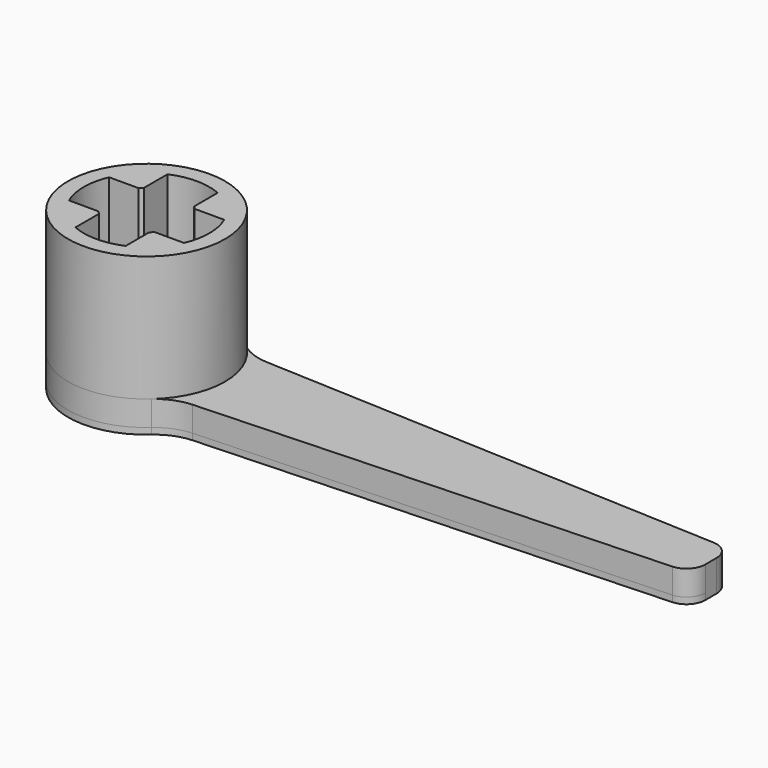
from build123d import *

# Parameters (mm, degrees)
F0_R     = 12.5
F1_DEPTH = 20
F3_DEPTH = 5
F4_DEPTH = 4
F5_R     = 8
F6_R     = 3


with BuildPart() as f1:
    # F0 (on Top) → F1 (new body)
    with BuildSketch(Plane.XY):
        Circle(F0_R)
        with BuildLine():
            ThreePointArc((-9.1651513899, -4), (-10, 0), (-9.1651513899, 4))
            Line((-9.1651513899, 4), (-4.472135955, 4))
            ThreePointArc((-4.472135955, 4), (-4.2426406871, 4.2426406871), (-4, 4.472135955))
            Line((-4, 4.472135955), (-4, 9.1651513899))
            ThreePointArc((-4, 9.1651513899), (0, 10), (4, 9.1651513899))
            Line((4, 9.1651513899), (4, 4.472135955))
            ThreePointArc((4, 4.472135955), (4.2426406871, 4.2426406871), (4.472135955, 4))
            Line((4.472135955, 4), (9.1651513899, 4))
            ThreePointArc((9.1651513899, 4), (10, 0), (9.1651513899, -4))
            Line((9.1651513899, -4), (4.472135955, -4))
            ThreePointArc((4.472135955, -4), (4.2426406871, -4.2426406871), (4, -4.472135955))
            Line((4, -4.472135955), (4, -9.1651513899))
            ThreePointArc((4, -9.1651513899), (0, -10), (-4, -9.1651513899))
            Line((-4, -9.1651513899), (-4, -4.472135955))
            ThreePointArc((-4, -4.472135955), (-4.2426406871, -4.2426406871), (-4.472135955, -4))
            Line((-4.472135955, -4), (-9.1651513899, -4))
        make_face(mode=Mode.SUBTRACT)
    extrude(amount=F1_DEPTH)

    # F2 (on Top) → F3 (join)
    with BuildSketch(Plane.XY):
        with BuildLine():
            ThreePointArc((10, -7.5), (11.8585412256, -3.9528470752), (12.5, 0))
            ThreePointArc((12.5, 0), (11.8585412256, 3.9528470752), (10, 7.5))
            ThreePointArc((10, 7.5), (-12.5, 0), (10, -7.5))
        make_face()
        with BuildLine():
            ThreePointArc((10, 7.5), (11.8585412256, 3.9528470752), (12.5, 0))
            ThreePointArc((12.5, 0), (11.8585412256, -3.9528470752), (10, -7.5))
            Line((10, -7.5), (89.9234008285, -4))
            Line((89.9234008285, -4), (89.9234008285, 0))
            Line((89.9234008285, 0), (89.9234008285, 4))
            Line((89.9234008285, 4), (10, 7.5))
        make_face()
    extrude(amount=-F3_DEPTH)

    # F2 (on Top) → F4 (join)
    with BuildSketch(Plane.XY):
        with BuildLine():
            ThreePointArc((10, -7.5), (11.8585412256, -3.9528470752), (12.5, 0))
            ThreePointArc((12.5, 0), (11.8585412256, 3.9528470752), (10, 7.5))
            ThreePointArc((10, 7.5), (-12.5, 0), (10, -7.5))
        make_face()
        with BuildLine():
            ThreePointArc((10, 7.5), (11.8585412256, 3.9528470752), (12.5, 0))
            ThreePointArc((12.5, 0), (11.8585412256, -3.9528470752), (10, -7.5))
            Line((10, -7.5), (89.9234008285, -4))
            Line((89.9234008285, -4), (89.9234008285, 0))
            Line((89.9234008285, 0), (89.9234008285, 4))
            Line((89.9234008285, 4), (10, 7.5))
        make_face()
    extrude(amount=-F4_DEPTH)

    # F5
    f5_edges = [f1.edges().sort_by_distance(p)[0] for p in [
        (10, 7.5, -2.5),
        (10, -7.5, -2.5),
    ]]
    fillet(f5_edges, radius=F5_R)

    # F6
    f6_edges = [f1.edges().sort_by_distance(p)[0] for p in [
        (89.923401, 4, -2.5),
        (89.923401, -4, -2.5),
    ]]
    fillet(f6_edges, radius=F6_R)


solid = f1.part
